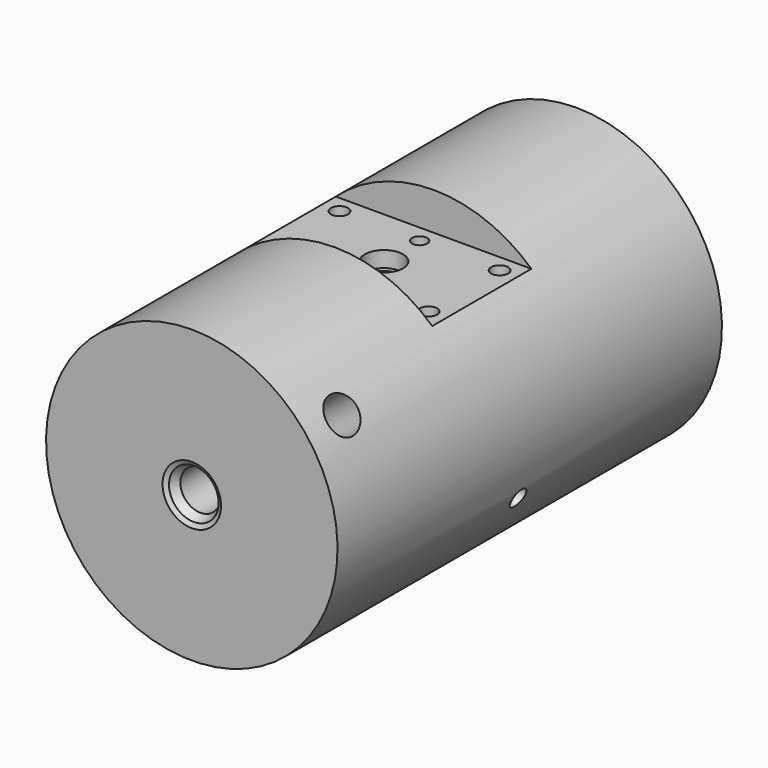
from build123d import *

# Parameters (mm, degrees)
F3_W            = 97.5
F3_H            = 59.3
F4_DEPTH        = 200
F6_D            = 45
F6_DEPTH        = 170
F6_CBORE_D      = 60
F6_CBORE_DEPTH  = 25
F6_TIP          = 13.5193639281
F7_D            = 24
F7_DEPTH        = 45
F7_TIP          = 7.2103274283
F8_D            = 27
F8_DEPTH        = 89
F8_TIP          = 8.1116183569
F13_D           = 30
F13_DEPTH       = 229
F13_TIP         = 9.0129092854
F18_D           = 58
F18_DEPTH       = 229
F18_TIP         = 17.4249579518
F23_D           = 38
F23_DEPTH       = 254
F23_TIP         = 11.4163517615
F24_D           = 38
F24_DEPTH       = 50
F24_TIP         = 11.4163517615
F26_D           = 16
F26_DEPTH       = 30
F26_TIP         = 4.8068849522
F27_D           = 36
F27_DEPTH       = 394
F27_CSINK_D     = 40
F27_CSINK_ANGLE = 60
F27_TIP         = 10.8154911425


# Not quite as in the source:
# - a pattern or mirror of a feature is missing from the dataset's text; its kind, count and spacing are read off the source's solid


with BuildPart() as f2:
    # F1 (on Right) → F2 (revolve)
    with BuildSketch(Plane.YZ):
        Polygon((0, 229.3), (0, 46), (4, 39), (16.9903810568, 31.5), (739.0096189432, 31.5), (752, 39), (756, 46), (756, 229.3), (378, 229.3), align=None)
    revolve(axis=Axis((0, 378, 0), (0, 1, 0)))

    # F3 (on Right) → F4 (cut, symmetric)
    with BuildSketch(Plane.YZ):
        with Locations((329.25, 199.65)):
            Rectangle(F3_W, F3_H)
        with Locations((426.75, 199.65)):
            Rectangle(F3_W, F3_H)
    extrude(amount=F4_DEPTH, both=True, mode=Mode.SUBTRACT)

    # F6
    with Locations(Plane.XY.offset(170)):
        with Locations((0, 378)):
            CounterBoreHole(F6_D / 2, F6_CBORE_D / 2, F6_CBORE_DEPTH, depth=F6_DEPTH)
            with Locations((0, 0, -(F6_DEPTH + F6_TIP / 2))):  # 118° drill point
                Cone(0, F6_D / 2, F6_TIP, mode=Mode.SUBTRACT)

    # F7
    with Locations(Plane.XY.offset(170)):
        with Locations((0, 308), (0, 448)):
            Hole(F7_D / 2, depth=F7_DEPTH)
            with Locations((0, 0, -(F7_DEPTH + F7_TIP / 2))):  # 118° drill point
                Cone(0, F7_D / 2, F7_TIP, mode=Mode.SUBTRACT)

    # F8
    with Locations(Plane.XY.offset(170)):
        with Locations((-126, 308), (-126, 448), (126, 448), (126, 308)):
            Hole(F8_D / 2, depth=F8_DEPTH)
            with Locations((0, 0, -(F8_DEPTH + F8_TIP / 2))):  # 118° drill point
                Cone(0, F8_D / 2, F8_TIP, mode=Mode.SUBTRACT)

    # F13
    with Locations(Plane(origin=(211.0717628966, 0, -89.5946477626), x_dir=(0, 1, 0), z_dir=(0.9205048535, 0, -0.3907311285))):
        with Locations((378, 0)):
            f13 = Hole(F13_D / 2, depth=F13_DEPTH)
            with Locations((0, 0, -(F13_DEPTH + F13_TIP / 2))):  # 118° drill point
                Cone(0, F13_D / 2, F13_TIP, mode=Mode.SUBTRACT)

    # F13_copies: F13 across plane
    add(f13.mirror(Plane(origin=(0.000261, 0, 0), x_dir=(-1e-06, 0, -1), z_dir=(-1, 0, 1e-06))), mode=Mode.SUBTRACT)

    # F18
    with Locations(Plane(origin=(180.690865802, 0, 141.1711762922), x_dir=(0, 1, 0), z_dir=(0.7880107536, 0, 0.6156614753))):
        with Locations((70, 0)):
            Hole(F18_D / 2, depth=F18_DEPTH)
            with Locations((0, 0, -(F18_DEPTH + F18_TIP / 2))):  # 118° drill point
                Cone(0, F18_D / 2, F18_TIP, mode=Mode.SUBTRACT)

    # F23 (one way)
    with BuildSketch(Plane(origin=(-206.1946202576, 0, 66.9966933789), x_dir=(0, 1, 0), z_dir=(-0.9510565163, 0, 0.3090169944))):
        with Locations((686, -74.657294708)):
            Circle(F23_D / 2)
    extrude(amount=-F23_DEPTH, mode=Mode.SUBTRACT)
    with Locations(Plane(origin=(-206.1946202576, 0, 66.9966933789), x_dir=(0, 1, 0), z_dir=(-0.9510565163, 0, 0.3090169944))):
        with Locations((686, -74.657294708)):
            with Locations((0, 0, -(F23_DEPTH + F23_TIP / 2))):  # 118° drill point
                Cone(0, F23_D / 2, F23_TIP, mode=Mode.SUBTRACT)

    # F24 (one way)
    with BuildSketch(Plane(origin=(-206.1946202576, 0, 66.9966933789), x_dir=(0, 1, 0), z_dir=(0.9510565163, 0, -0.3090169944))):
        with Locations((686, 74.657294708)):
            Circle(F24_D / 2)
    extrude(amount=-F24_DEPTH, mode=Mode.SUBTRACT)
    with Locations(Plane(origin=(-206.1946202576, 0, 66.9966933789), x_dir=(0, 1, 0), z_dir=(0.9510565163, 0, -0.3090169944))):
        with Locations((686, 74.657294708)):
            with Locations((0, 0, -(F24_DEPTH + F24_TIP / 2))):  # 118° drill point
                Cone(0, F24_D / 2, F24_TIP, mode=Mode.SUBTRACT)

    # F26
    with Locations(Plane(origin=(0, 756, 0), x_dir=(-1, 0, 0), z_dir=(0, 1, 0))):
        with Locations((0, 115), (0, -115)):
            Hole(F26_D / 2, depth=F26_DEPTH)
            with Locations((0, 0, -(F26_DEPTH + F26_TIP / 2))):  # 118° drill point
                Cone(0, F26_D / 2, F26_TIP, mode=Mode.SUBTRACT)

    # F27
    with Locations(Plane(origin=(0, 756, 0), x_dir=(-1, 0, 0), z_dir=(0, 1, 0))):
        with Locations((-49, 80), (49, 80)):
            CounterSinkHole(F27_D / 2, F27_CSINK_D / 2, depth=F27_DEPTH, counter_sink_angle=F27_CSINK_ANGLE)
            with Locations((0, 0, -(F27_DEPTH + F27_TIP / 2))):  # 118° drill point
                Cone(0, F27_D / 2, F27_TIP, mode=Mode.SUBTRACT)


solid = f2.part
